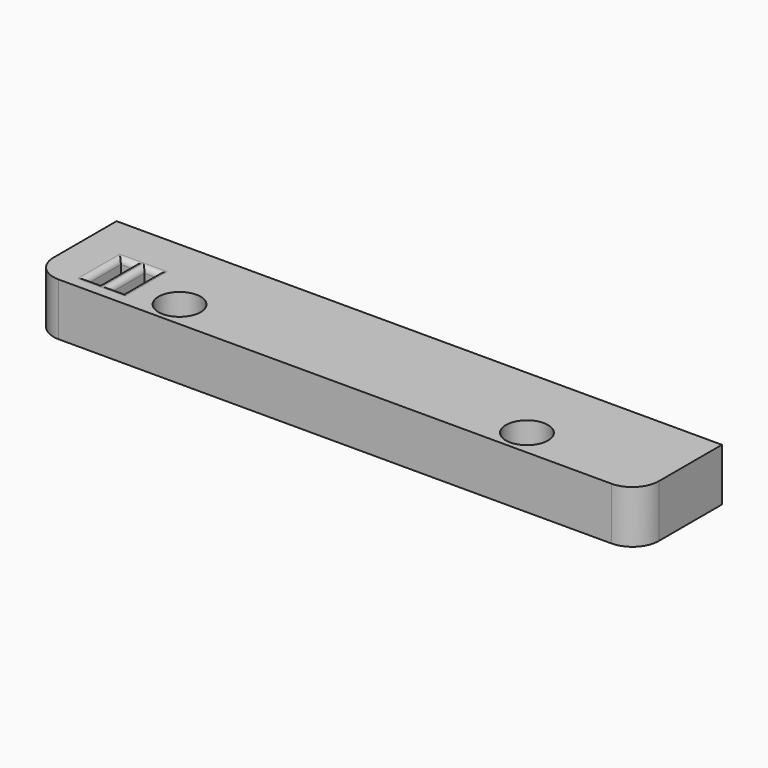
from build123d import *

# Parameters (mm, degrees)
F0_W     = 115
F0_H     = 20
F1_DEPTH = 10
F2_R     = 4
F3_DEPTH = 8
F4_R     = 1.5
F5_DEPTH = 12
F6_R     = 5
F7_W     = 2.5
F7_H     = 8
F8_DEPTH = 25
F9_R     = 0.99999


# Not quite as in the source:
# - a fillet or chamfer is up to 0.001 mm smaller than in the source, because OpenCascade refuses the exact size


with BuildPart() as f1:
    # F0 (on Top) → F1 (new body)
    with BuildSketch(Plane.XY):
        with Locations((-1.558380723, -11.7337754572)):
            Rectangle(F0_W, F0_H)
    extrude(amount=F1_DEPTH)

    # F2 (on face) → F3 (cut)
    with BuildSketch(Plane.XY.offset(10)):
        with Locations((-35.058380723, -16.7792532593)):
            Circle(F2_R)
        with Locations((30.941619277, -16.7792532593)):
            Circle(F2_R)
    extrude(amount=-F3_DEPTH, mode=Mode.SUBTRACT)

    # F4 (on face) → F5 (cut)
    with BuildSketch(Plane(origin=(0, -1.7337754572, 0), x_dir=(-1, 0, 0), z_dir=(0, 1, 0))):
        with Locations((54.058380723, 6.6987262902)):
            Circle(F4_R)
        with Locations((-49.941619277, 6.6987262902)):
            Circle(F4_R)
    extrude(amount=-F5_DEPTH, mode=Mode.SUBTRACT)

    # F6
    f6_edges = [f1.edges().sort_by_distance(p)[0] for p in [
        (-59.058381, -21.733775, 5),
        (55.941619, -21.733775, 5),
    ]]
    fillet(f6_edges, radius=F6_R)

    # F7 (on face) → F8 (cut)
    with BuildSketch(Plane.XY.offset(10)):
        with Locations((-49.808380723, -14.7337754572)):
            Rectangle(F7_W, F7_H)
        with Locations((-45.308380723, -14.7337754572)):
            Rectangle(F7_W, F7_H)
    extrude(amount=-F8_DEPTH, mode=Mode.SUBTRACT)

    # F9 (radius 1 in the source; OpenCascade refuses exactly that, so slightly less here)
    f9_edges = [f1.edges().sort_by_distance(p)[0] for p in [
        (-51.058381, -14.733775, 10),
        (-49.808381, -10.733775, 10),
        (-48.558381, -14.733775, 10),
        (-49.808381, -18.733775, 10),
        (-45.308381, -18.733775, 10),
        (-46.558381, -14.733775, 10),
        (-45.308381, -10.733775, 10),
        (-44.058381, -14.733775, 10),
        (-44.058381, -14.733775, 0),
        (-45.308381, -10.733775, 0),
        (-46.558381, -14.733775, 0),
        (-45.308381, -18.733775, 0),
        (-49.808381, -18.733775, 0),
        (-48.558381, -14.733775, 0),
        (-49.808381, -10.733775, 0),
        (-51.058381, -14.733775, 0),
    ]]
    fillet(f9_edges, radius=F9_R)


solid = f1.part
